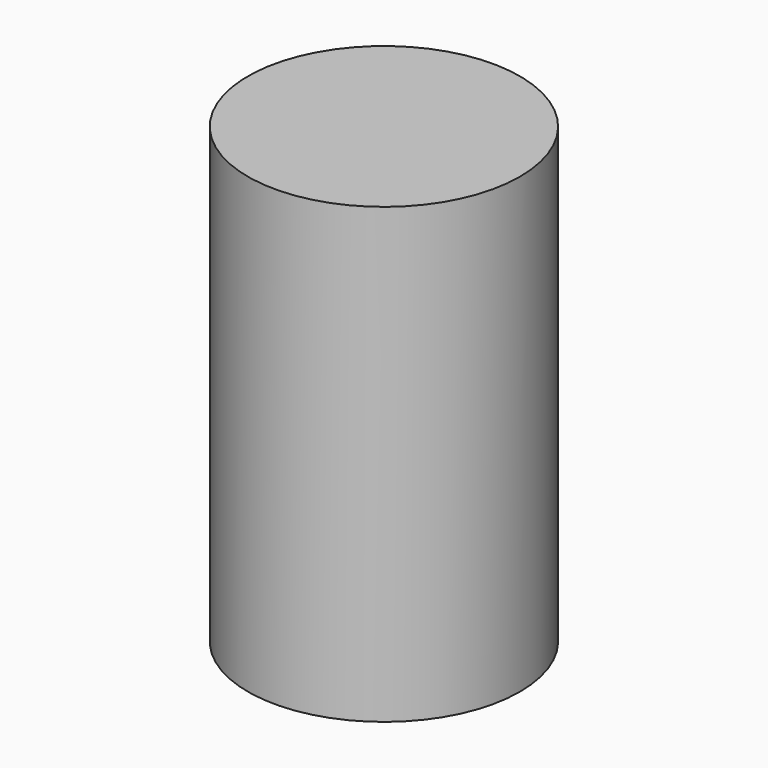
from build123d import *

# Parameters (mm, degrees)
F0_R     = 30
F1_DEPTH = 50
F2_T     = -1
F3_R     = 30
F4_DEPTH = 1


with BuildPart() as f1:
    # F0 (on Top) → F1 (new body, symmetric)
    with BuildSketch(Plane.XY):
        Circle(F0_R)
    extrude(amount=F1_DEPTH, both=True)

    # F2
    f2_openings = [f1.faces().sort_by_distance(p)[0] for p in [
        (0, 0, 50),
    ]]
    offset(amount=F2_T, openings=f2_openings)

    # F3 (on face) → F4 (join)
    with BuildSketch(Plane.XY.offset(50)):
        Circle(F3_R)
    extrude(amount=-F4_DEPTH)


solid = f1.part
